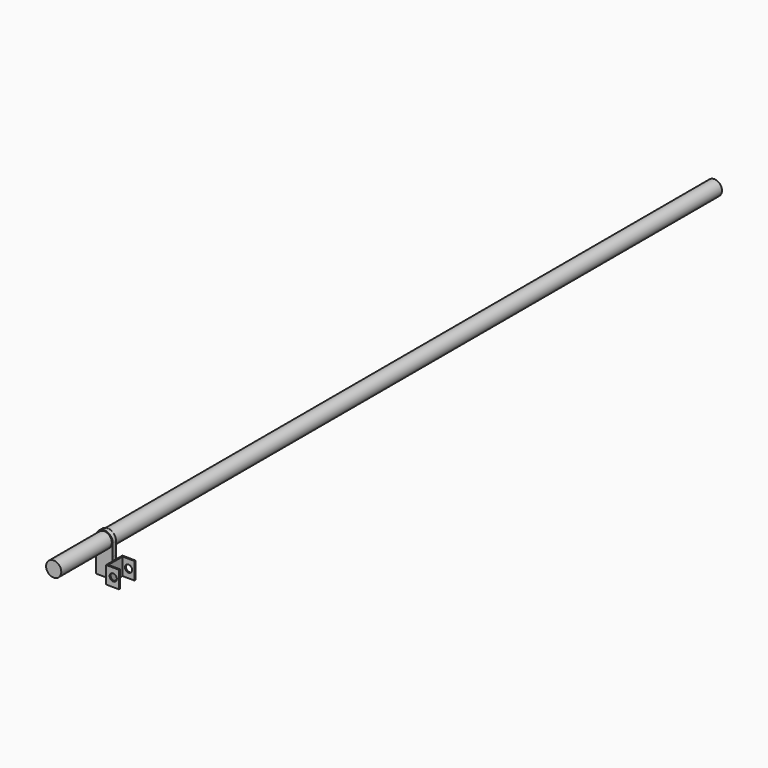
from build123d import *

# Parameters (mm, degrees)
F1_DEPTH      = 1.27
F2_R          = 2.2887754184
F3_DEPTH      = 228.6
F3_DEPTH_BACK = 20.32
F4_W          = 1.27
F4_H          = 3.4091206923
F5_DEPTH      = 3.937
F6_T          = -0.381
F7_R          = 1.080450049
F8_DEPTH      = 11.176


# Not quite as in the source:
# - a feature names something its author has since deleted; it is built from what else it names


with BuildPart() as f1:
    # F0 (on Front) → F1 (new body)
    with BuildSketch(Plane.XZ):
        with BuildLine():
            ThreePointArc((-2.5559609307, 5.4012401961), (0, 2.8452792654), (2.5559609307, 5.4012401961))
            ThreePointArc((2.5559609307, 5.4012401961), (0, 7.9572011268), (-2.5559609307, 5.4012401961))
        make_face()
        with BuildLine():
            Line((2.5559609307, 1.721014436), (2.5559609307, 5.4012401961))
            ThreePointArc((2.5559609307, 5.4012401961), (0, 2.8452792654), (-2.5559609307, 5.4012401961))
            Line((-2.5559609307, 5.4012401961), (-2.5559609307, 4.3758706689))
            Line((-2.5559609307, 4.3758706689), (-2.5559609307, -2.8266729787))
            Line((-2.5559609307, -2.8266729787), (-2.5559609307, -4.3681138195))
            Line((-2.5559609307, -4.3681138195), (2.5204877513, -4.3681138195))
            Line((2.5204877513, -4.3681138195), (2.5204877513, -2.8266729787))
            Line((2.5204877513, -2.8266729787), (2.5559609307, 1.721014436))
        make_face()
    extrude(amount=-F1_DEPTH)

    # F2 (on face) → F3 (join, two sides)
    with BuildSketch(Plane(origin=(0, 1.27, 0), x_dir=(-1, 0, 0), z_dir=(0, 1, 0))) as f3_sk:
        with Locations((0, 5.4012401961)):
            Circle(F2_R)
    extrude(amount=F3_DEPTH)
    extrude(f3_sk.sketch, amount=-F3_DEPTH_BACK)


with BuildPart() as f5:
    # F4 (on face) → F5 (new body)
    with BuildSketch(Plane(origin=(2.5423818682, 0, -0.0198312593), x_dir=(0, 1, 0), z_dir=(0.9999695793, 0, -0.0078000304))):
        Polygon((-2.497356755, -4.576918826), (3.6564493494, -4.576918826), (3.6564493494, 0.6021935842), (1.27, 0.6021935842), (1.27, -2.8069271081), (0, -2.8069271081), (0, 0.6021935842), (-2.497356755, 0.6021935842), align=None)
        with Locations((0.635, -1.102366762)):
            Rectangle(F4_W, F4_H)
    extrude(amount=F5_DEPTH)

    # F6
    f6_openings = [f5.faces().sort_by_distance(p)[0] for p in [
        (6.463761, 0.579546, -2.037842),
        (4.515519, 0.579546, 0.56699),
        (4.475122, 0.579546, -4.611965),
    ]]
    offset(amount=F6_T, openings=f6_openings)

    # F7 (on face) → F8 (cut)
    with BuildSketch(Plane.XZ.offset(2.497356755)):
        with Locations((4.7060133182, -2.0378421431)):
            Circle(F7_R)
    extrude(amount=-F8_DEPTH, mode=Mode.SUBTRACT)


solid = Compound([f1.part, f5.part])
